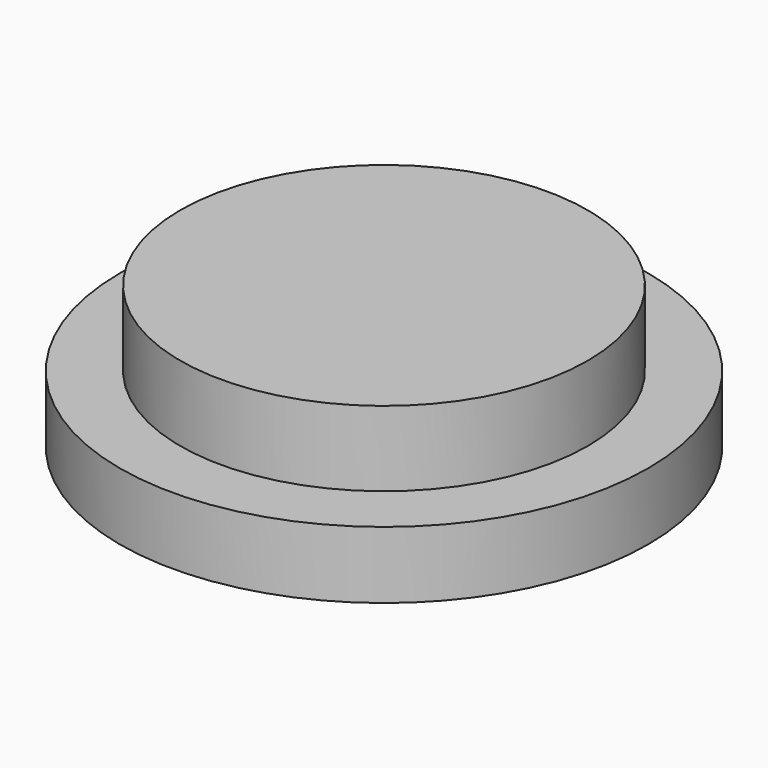
from build123d import *

# Parameters (mm, degrees)
F0_R     = 98.5012
F0_R_2   = 75.9968
F1_DEPTH = 24.9936
F2_DEPTH = 53.0098


# Not quite as in the source:
# - a feature names something its author has since deleted; it is built from what else it names
# - the program builds the solid bodies; features that only make, move or delete a surface that nothing else refers to are left out


with BuildPart() as f1:
    # F0 (on Top) → F1 (new body)
    with BuildSketch(Plane.XY):
        Circle(F0_R)
        Circle(F0_R_2, mode=Mode.SUBTRACT)
    extrude(amount=F1_DEPTH)

    # F0 (on Top) → F2 (join)
    with BuildSketch(Plane.XY):
        Circle(F0_R_2)
    extrude(amount=F2_DEPTH)


solid = f1.part
